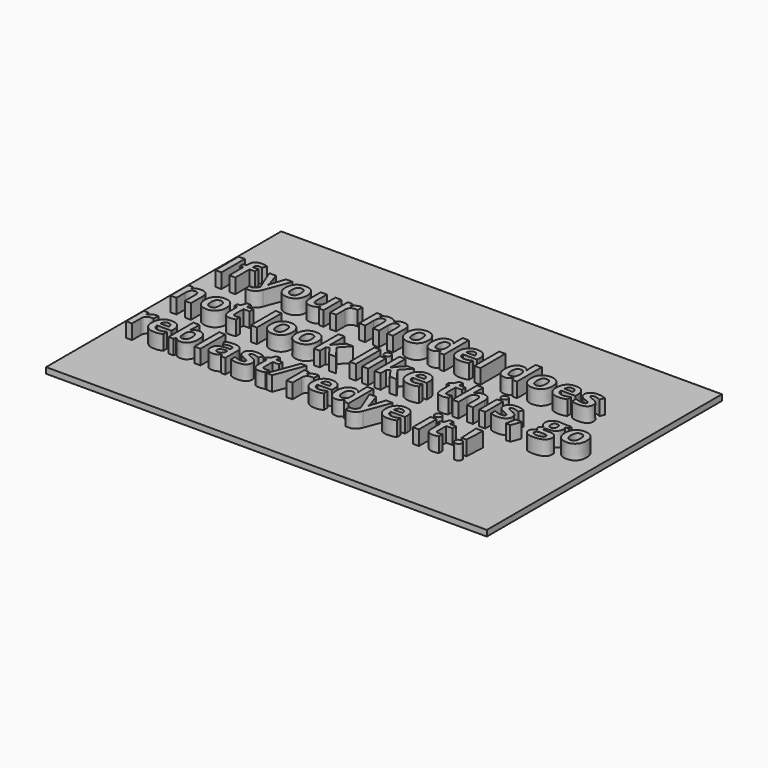
from build123d import *

# Parameters (mm, degrees)
F0_W         = 150
F0_H         = 100
F2_DEPTH     = 2
F1_TEXT_SIZE = 13.8888888889
F3_DEPTH     = 5


# Not quite as in the source:
# - Text() gives the source's letters only with a copy of the font that has no kerning and outlines rounded to 1/6400 em; it was checked with that copy


with BuildPart() as f2:
    # F0 (on Top) → F2 (new body)
    with BuildSketch(Plane.XY):
        Rectangle(F0_W, F0_H)
    extrude(amount=-F2_DEPTH)

    # F1 (on Top) → F3 (join)
    with BuildSketch(Plane.XY):
        with Locations((-70.0100871172, 14.1727423113)):
            Text('If your model does', F1_TEXT_SIZE, font='Open Sans', font_style=FontStyle.BOLD, text_align=(TextAlign.LEFT, TextAlign.BOTTOM))
        with Locations((-70.0100871172, -4.7161465776)):
            Text('not look like this, go', F1_TEXT_SIZE, font='Open Sans', font_style=FontStyle.BOLD, text_align=(TextAlign.LEFT, TextAlign.BOTTOM))
        with Locations((-70.0100871172, -23.6050354665)):
            Text('reblast/redye it !', F1_TEXT_SIZE, font='Open Sans', font_style=FontStyle.BOLD, text_align=(TextAlign.LEFT, TextAlign.BOTTOM))
    extrude(amount=F3_DEPTH)


solid = f2.part
